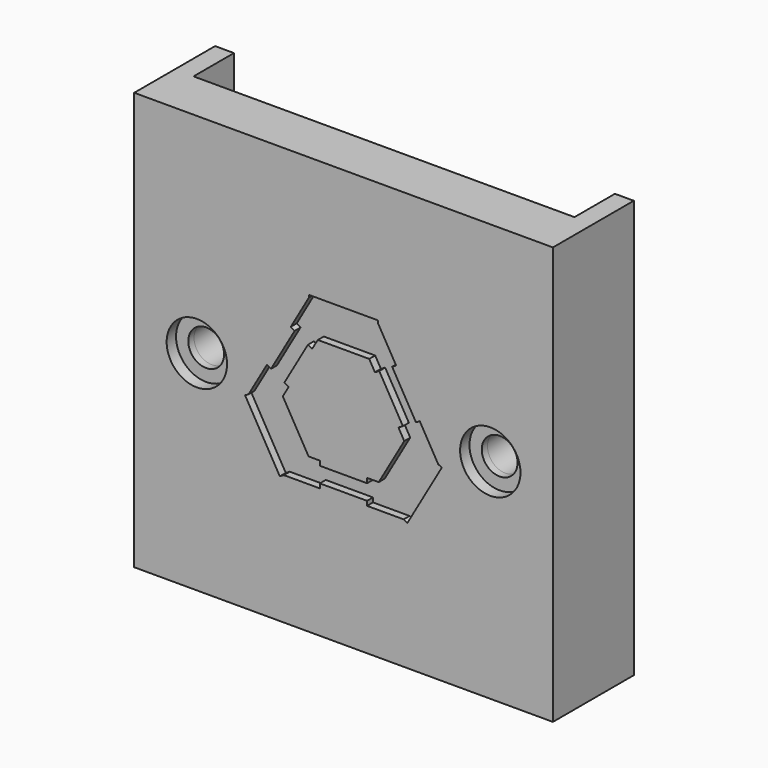
from build123d import *
from build123d import SkipClean  # not in build123d's __all__

# Parameters (mm, degrees)
F1_DEPTH  = 24.13
F2_R      = 2.032
F2_R_2    = 1.2065
F3_DEPTH  = 0.7874
F4_DEPTH  = 25.4
F6_DEPTH  = 0.5
F7_DEPTH  = 2
F8_DEPTH  = 2
F9_W      = 25.654
F9_H      = 1
F10_DEPTH = 1.27
F11_R     = 1.2065
F12_DEPTH = 1.905
F13_DEPTH = 1.905
F14_DEPTH = 1.0414


# Not quite as in the source:
# - after a boolean that leaves OpenCascade's solid faulty, fix() repairs it
# - a feature names something its author has since deleted; it is built from what else it names


with BuildPart() as f1:
    # F0 (on Top) → F1 (new body)
    with BuildSketch(Plane.XY):
        Polygon((-22.881621525, -1.6067087497), (-22.881621525, 2.0254912503), (-24.151621525, 2.0254912503), (-24.151621525, -2.8767087497), (4.042378475, -2.8767087497), (4.042378475, 2.0254912503), (2.772378475, 2.0254912503), (2.772378475, -1.6067087497), align=None)
    extrude(amount=F1_DEPTH)

    # F2 (on face) → F3 (cut)
    with BuildSketch(Plane.XZ.offset(2.8767087497)):
        with Locations((-19.935221525, 12.065)):
            Circle(F2_R)
        with Locations((-19.935221525, 12.065)):
            Circle(F2_R_2, mode=Mode.SUBTRACT)
        with Locations((-0.174021525, 12.065)):
            Circle(F2_R)
        with Locations((-0.174021525, 12.065)):
            Circle(F2_R_2, mode=Mode.SUBTRACT)
    extrude(amount=-F3_DEPTH, mode=Mode.SUBTRACT)

    # F4 (cut): faces of the model
    f4_faces = [f1.faces().sort_by_distance(p)[0] for p in [
        (-19.935221525, -2.8767087497, 12.065),
        (-0.174021525, -2.8767087497, 12.065),
    ]]
    extrude(f4_faces, amount=-F4_DEPTH, mode=Mode.SUBTRACT)

    # F5 (on face) → F6 (cut)
    with BuildSketch(Plane.XZ.offset(2.8767087497)):
        Polygon((-12.3912415756, 17.8113617003), (-13.6065593278, 15.684556216), (-13.3501001609, 15.5277705701), (-14.9427792273, 12.7550959473), (-15.21558023, 12.9117982314), (-16.4524054843, 10.7586249602), (-16.6849697297, 10.6241926551), (-14.3470017528, 6.5795714036), (-14.0742704561, 6.7396221901), (-11.6537952153, 6.7396221901), (-11.6537952153, 7.0368205197), (-8.471750264, 7.0368205197), (-8.471750264, 6.7396221901), (-6.0077723583, 6.7396221901), (-5.7620638571, 6.5984823741), (-3.4414858846, 10.6383468956), (-3.6771140247, 10.7619399543), (-4.9225916905, 12.9113931759), (-5.1792576933, 12.7626708074), (-6.7848130465, 15.533548376), (-6.5128039159, 15.6911611557), (-7.7413314311, 17.8113617003), (-7.7413314311, 17.9749652743), (-12.3912415756, 17.9749652743), align=None)
        Polygon((-12.1788967651, 14.8354667667), (-11.7852579159, 15.4973436147), (-8.3281154101, 15.4973436147), (-7.9414616069, 14.830054039), (-7.6521674377, 14.9976824493), (-6.0583813106, 12.2471162856), (-6.3580625964, 12.0734691718), (-5.9656283895, 11.396203739), (-7.6865507823, 8.4002719491), (-8.471750264, 8.4002719491), (-8.471750264, 8.0795111135), (-11.6385354949, 8.0795111135), (-11.6385354949, 8.3887251094), (-12.4105562744, 8.3887251094), (-14.1476861274, 11.3866747806), (-13.7563398992, 12.0679644255), (-14.0430930461, 12.2326810967), (-12.4564279131, 14.9948861397), align=None, mode=Mode.SUBTRACT)
    extrude(amount=-F6_DEPTH, mode=Mode.SUBTRACT)

    # F7 (add): a face of the model
    f7_faces = [f1.faces().sort_by_distance(p)[0] for p in [
        (-10.054621525, -1.7395492941, 0),
    ]]
    extrude(f7_faces, amount=F7_DEPTH)

    # F8 (add): a face of the model
    f8_faces = [f1.faces().sort_by_distance(p)[0] for p in [
        (-10.054621525, -1.7395492941, 24.13),
    ]]
    extrude(f8_faces, amount=F8_DEPTH)

    # F9 (on face) → F10 (join)
    with BuildSketch(Plane(origin=(0, -1.6067087497, 0), x_dir=(-1, 0, 0), z_dir=(0, 1, 0))):
        with Locations((10.054621525, 25.63)):
            Rectangle(F9_W, F9_H)
        with Locations((10.054621525, -1.5)):
            Rectangle(F9_W, F9_H)
    extrude(amount=F10_DEPTH)

    # F11 (on face) → F12 (join)
    with BuildSketch(Plane(origin=(0, -1.6067087497, 0), x_dir=(-1, 0, 0), z_dir=(0, 1, 0))):
        with BuildLine():
            ThreePointArc((-2.772378475, 6.4958446701), (-1.4028429606, 8.7376625106), (0.8266095876, 10.1272365784))
            ThreePointArc((0.8266095876, 10.1272365784), (2.218721566, 12.065), (0.8266095876, 14.0027634216))
            ThreePointArc((0.8266095876, 14.0027634216), (-1.4028429606, 15.3923374894), (-2.772378475, 17.6341553299))
            Line((-2.772378475, 17.6341553299), (-2.772378475, 6.4958446701))
        make_face()
        with Locations((0.174021525, 12.065)):
            Circle(F11_R, mode=Mode.SUBTRACT)
        with BuildLine():
            ThreePointArc((19.2826334624, 10.1272365784), (21.5120860106, 8.7376625106), (22.881621525, 6.4958446701))
            Line((22.881621525, 6.4958446701), (22.881621525, 17.6341553299))
            ThreePointArc((22.881621525, 17.6341553299), (21.5120860106, 15.3923374894), (19.2826334624, 14.0027634216))
            ThreePointArc((19.2826334624, 14.0027634216), (17.890521484, 12.065), (19.2826334624, 10.1272365784))
        make_face()
        with Locations((19.935221525, 12.065)):
            Circle(F11_R, mode=Mode.SUBTRACT)
    with SkipClean():  # cleaning this boolean's faces spoils the solid; the shape is the same uncleaned
        extrude(amount=F12_DEPTH)

    # F13 (add): faces of the model
    f13_faces = [f1.faces().sort_by_distance(p)[0] for p in [
        (-23.516621525, 2.0254912503, 12.065),
        (-10.054621525, -0.3367087497, 25.63),
        (-10.054621525, -0.3367087497, -1.5),
        (3.407378475, 2.0254912503, 12.065),
    ]]
    extrude(f13_faces, amount=F13_DEPTH)

    add(f1.part.fix(), mode=Mode.REPLACE)

    # F14 (cut): a face of the model
    f14_faces = [f1.faces().sort_by_distance(p)[0] for p in [
        (-10.054621525, 1.5682912503, 25.63),
    ]]
    extrude(f14_faces, amount=-F14_DEPTH, mode=Mode.SUBTRACT)


solid = f1.part
